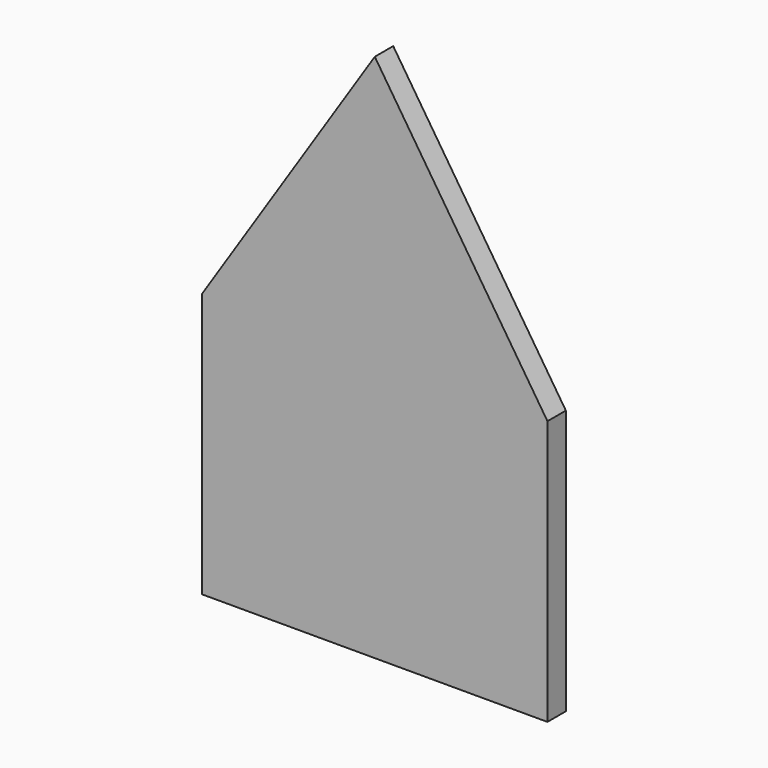
from build123d import *

# Parameters (mm, degrees)
F1_DEPTH = 2


with BuildPart() as f1:
    # F0 (on Front) → F1 (new body)
    with BuildSketch(Plane.XZ):
        Polygon((0, -11.5), (15, -11.5), (15, 11.5), (0, 34.5), align=None)
        Polygon((-15, -11.5), (0, -11.5), (0, 34.5), (-15, 11.5), align=None)
    extrude(amount=F1_DEPTH)


solid = f1.part
